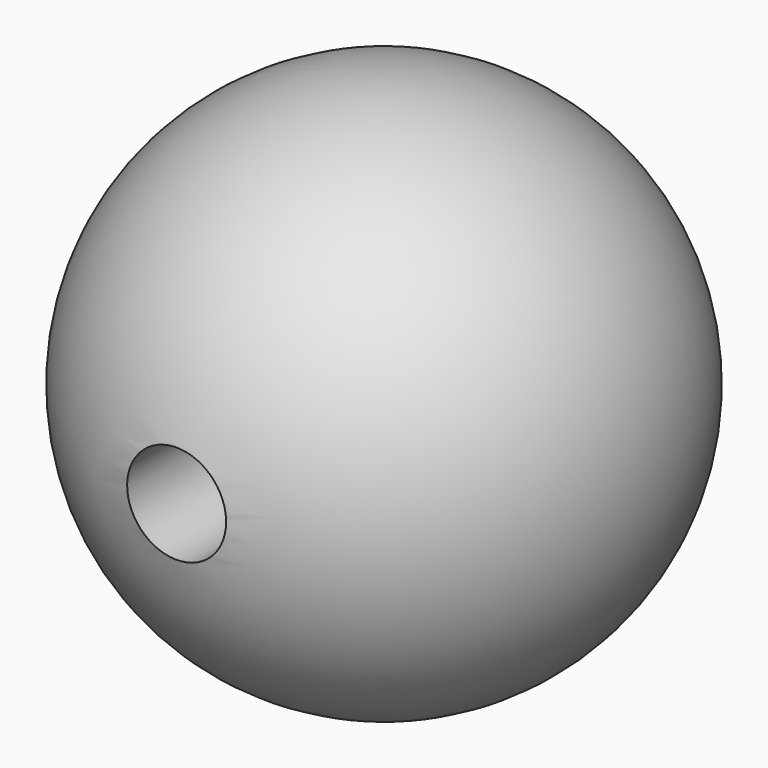
from build123d import *

# Parameters (mm, degrees)
F2_D     = 9.525
F2_DEPTH = 25.401


# Not quite as in the source:
# - a feature names something its author has since deleted; it is built from what else it names


with BuildPart() as f1:
    # F0 (on Front) → F1 (revolve)
    with BuildSketch(Plane.XZ):
        with BuildLine():
            Line((0, -25.4), (0, 25.4))
            ThreePointArc((0, 25.4), (-25.4, 0), (0, -25.4))
        make_face()
    revolve(axis=Axis((0, 0, 0), (0, 0, -1)))

    # F2 (through all, one way)
    with BuildSketch(Plane(origin=(0, 0, 0), x_dir=(1, 0, 0), z_dir=(0, 1, 0))):
        with Locations((0, 0)):
            Circle(F2_D / 2)
    extrude(amount=-F2_DEPTH, mode=Mode.SUBTRACT)


solid = f1.part
